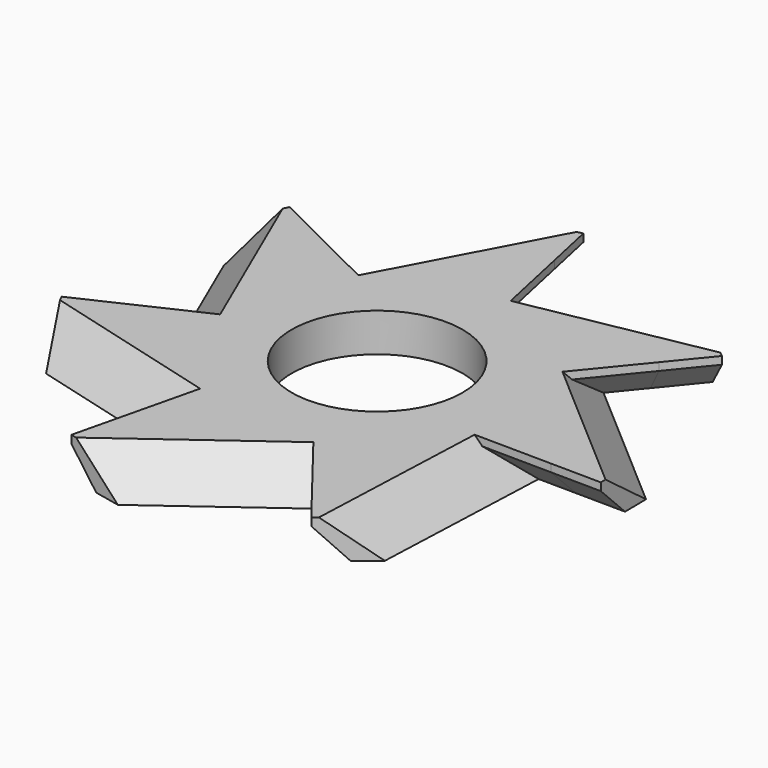
from build123d import *

# Parameters (mm, degrees)
F0_R         = 11.1
F1_DEPTH     = 5
F2_T4_DEPTH  = 66.9224244324
F2_T10_DEPTH = 66.9224244324
F2_T16_DEPTH = 66.9224244324
F2_T22_DEPTH = 66.9224244324
F2_T28_DEPTH = 66.9224244324
F2_T34_DEPTH = 66.9224244324
F2_T40_DEPTH = 66.9224244324
F3_SIZE      = 4


# Not quite as in the source:
# - a fillet or chamfer that OpenCascade refuses, or shapes differently, is made with other operations: its cross-section is extruded or revolved along the edge and cut away or added


with BuildPart() as f1:
    # F0 (on Top) → F1 (new body)
    with BuildSketch(Plane.XY):
        with BuildLine():
            ThreePointArc((13.9102940248, -6.3947663514), (14.9558155311, -3.2730564225), (15.3097784616, 0))
            ThreePointArc((15.3097784616, 0), (14.9174264356, 3.4437922532), (13.7604803953, 6.7110726292))
            ThreePointArc((13.7604803953, 6.7110726292), (13.7168049275, 6.7998955231), (13.6725561219, 6.8884341936))
            ThreePointArc((13.6725561219, 6.8884341936), (9.4080501116, 12.077992782), (3.3325913325, 14.9426621308))
            ThreePointArc((3.3325913325, 14.9426621308), (3.2359155889, 14.9638954436), (3.1391045899, 14.9845032923))
            ThreePointArc((3.1391045899, 14.9845032923), (-3.577131702, 14.8860150924), (-9.6048069761, 11.9221222731))
            ThreePointArc((-9.6048069761, 11.9221222731), (-9.6816841888, 11.8597768872), (-9.7581567243, 11.7969357838))
            ThreePointArc((-9.7581567243, 11.7969357838), (-13.8686603838, 6.4845644188), (-15.3095897294, -0.0760188232))
            ThreePointArc((-15.3095897294, -0.0760188232), (-15.308778302, -0.1749955606), (-15.307326995, -0.2739649836))
            ThreePointArc((-15.307326995, -0.2739649836), (-13.7168049275, -6.7998955231), (-9.4859391577, -12.0169161951))
            ThreePointArc((-9.4859391577, -12.0169161951), (-9.4080501116, -12.077992782), (-9.3297678259, -12.1385645305))
            ThreePointArc((-9.3297678259, -12.1385645305), (-3.2359155889, -14.9638954436), (3.4808170776, -14.9088305717))
            ThreePointArc((3.4808170776, -14.9088305717), (3.577131702, -14.8860150924), (3.6732968087, -14.8625774043))
            ThreePointArc((3.6732968087, -14.8625774043), (9.6816841888, -11.8597768872), (13.8264470578, -6.5740914431))
            ThreePointArc((13.8264470578, -6.5740914431), (13.8686603838, -6.4845644188), (13.9102940248, -6.3947663514))
        make_face()
        Circle(F0_R, mode=Mode.SUBTRACT)
        with BuildLine():
            ThreePointArc((13.6725561219, 6.8884341936), (13.7168049275, 6.7998955231), (13.7604803953, 6.7110726292))
            Line((13.7604803953, 6.7110726292), (28.1393743339, 1.1806929027))
            Line((28.1393743339, 1.1806929027), (27.8254993307, -6.5534854768))
            Line((27.8254993307, -6.5534854768), (34.3666750494, -6.6280952053))
            Line((34.3666750494, -6.6280952053), (34.1806906403, 7.5286378152))
            Line((34.1806906403, 7.5286378152), (22.47263633, 17.6688200307))
            Line((22.47263633, 17.6688200307), (13.6725561219, 6.8884341936))
        make_face()
        with BuildLine():
            ThreePointArc((13.7604803953, 6.7110726292), (14.9174264356, 3.4437922532), (15.3097784616, 0))
            ThreePointArc((15.3097784616, 0), (14.9558155311, -3.2730564225), (13.9102940248, -6.3947663514))
            Line((13.9102940248, -6.3947663514), (27.8254993307, -6.5534854768))
            Line((27.8254993307, -6.5534854768), (28.1393743339, 1.1806929027))
            Line((28.1393743339, 1.1806929027), (13.7604803953, 6.7110726292))
        make_face()
        with BuildLine():
            Line((27.8254993307, -6.5534854768), (13.9102940248, -6.3947663514))
            ThreePointArc((13.9102940248, -6.3947663514), (13.8686603838, -6.4845644188), (13.8264470578, -6.5740914431))
            Line((13.8264470578, -6.5740914431), (18.4677158103, -21.2640987672))
            Line((18.4677158103, -21.2640987672), (12.2251937987, -25.8408827536))
            Line((12.2251937987, -25.8408827536), (16.2452179168, -31.0014982676))
            Line((16.2452179168, -31.0014982676), (27.1974380987, -22.0295111355))
            Line((27.1974380987, -22.0295111355), (27.8254993307, -6.5534854768))
        make_face()
        with BuildLine():
            Line((18.4677158103, -21.2640987672), (13.8264470578, -6.5740914431))
            ThreePointArc((13.8264470578, -6.5740914431), (9.6816841888, -11.8597768872), (3.6732968087, -14.8625774043))
            Line((3.6732968087, -14.8625774043), (12.2251937987, -25.8408827536))
            Line((12.2251937987, -25.8408827536), (18.4677158103, -21.2640987672))
        make_face()
        with BuildLine():
            Line((12.2251937987, -25.8408827536), (3.6732968087, -14.8625774043))
            ThreePointArc((3.6732968087, -14.8625774043), (3.577131702, -14.8860150924), (3.4808170776, -14.9088305717))
            Line((3.4808170776, -14.9088305717), (-5.1105093912, -27.6965903568))
            Line((-5.1105093912, -27.6965903568), (-12.5809320123, -25.669568259))
            Line((-12.5809320123, -25.669568259), (-14.1092196492, -32.0301408191))
            Line((-14.1092196492, -32.0301408191), (-0.2660400579, -34.9989888809))
            Line((-0.2660400579, -34.9989888809), (12.2251937987, -25.8408827536))
        make_face()
        with BuildLine():
            Line((-5.1105093912, -27.6965903568), (3.4808170776, -14.9088305717))
            ThreePointArc((3.4808170776, -14.9088305717), (-3.2359155889, -14.9638954436), (-9.3297678259, -12.1385645305))
            Line((-9.3297678259, -12.1385645305), (-12.5809320123, -25.669568259))
            Line((-12.5809320123, -25.669568259), (-5.1105093912, -27.6965903568))
        make_face()
        with BuildLine():
            Line((-12.5809320123, -25.669568259), (-9.3297678259, -12.1385645305))
            ThreePointArc((-9.3297678259, -12.1385645305), (-9.4080501116, -12.077992782), (-9.4859391577, -12.0169161951))
            Line((-9.4859391577, -12.0169161951), (-24.8404167857, -13.2729845003))
            Line((-24.8404167857, -13.2729845003), (-27.9133594138, -6.1685453016))
            Line((-27.9133594138, -6.1685453016), (-33.8391270437, -8.939434038))
            Line((-33.8391270437, -8.939434038), (-27.5291846246, -21.6135141498))
            Line((-27.5291846246, -21.6135141498), (-12.5809320123, -25.669568259))
        make_face()
        with BuildLine():
            ThreePointArc((-15.307326995, -0.2739649836), (-15.308778302, -0.1749955606), (-15.3095897294, -0.0760188232))
            Line((-15.3095897294, -0.0760188232), (-25.8649836884, 11.1454494045))
            Line((-25.8649836884, 11.1454494045), (-22.2264578479, 17.9775180833))
            Line((-22.2264578479, 17.9775180833), (-28.0874815819, 20.8828489049))
            Line((-28.0874815819, 20.8828489049), (-34.062291676, 8.0473775715))
            Line((-34.062291676, 8.0473775715), (-27.9133594138, -6.1685453016))
            Line((-27.9133594138, -6.1685453016), (-15.307326995, -0.2739649836))
        make_face()
        with BuildLine():
            ThreePointArc((-15.3095897294, -0.0760188232), (-13.8686603838, 6.4845644188), (-9.7581567243, 11.7969357838))
            Line((-9.7581567243, 11.7969357838), (-22.2264578479, 17.9775180833))
            Line((-22.2264578479, 17.9775180833), (-25.8649836884, 11.1454494045))
            Line((-25.8649836884, 11.1454494045), (-15.3095897294, -0.0760188232))
        make_face()
        with BuildLine():
            ThreePointArc((-9.7581567243, 11.7969357838), (-9.6816841888, 11.8597768872), (-9.6048069761, 11.9221222731))
            Line((-9.6048069761, 11.9221222731), (-7.4126903243, 27.171132582))
            Line((-7.4126903243, 27.171132582), (0.1974198146, 28.5861436769))
            Line((0.1974198146, 28.5861436769), (-1.1853896087, 34.97992069))
            Line((-1.1853896087, 34.97992069), (-14.9457983513, 31.6484298448))
            Line((-14.9457983513, 31.6484298448), (-22.2264578479, 17.9775180833))
            Line((-22.2264578479, 17.9775180833), (-9.7581567243, 11.7969357838))
        make_face()
        with BuildLine():
            ThreePointArc((-9.6048069761, 11.9221222731), (-3.577131702, 14.8860150924), (3.1391045899, 14.9845032923))
            Line((3.1391045899, 14.9845032923), (0.1974198146, 28.5861436769))
            Line((0.1974198146, 28.5861436769), (-7.4126903243, 27.171132582))
            Line((-7.4126903243, 27.171132582), (-9.6048069761, 11.9221222731))
        make_face()
        with BuildLine():
            ThreePointArc((3.1391045899, 14.9845032923), (3.2359155889, 14.9638954436), (3.3325913325, 14.9426621308))
            Line((3.3325913325, 14.9426621308), (16.6215100454, 22.7363987351))
            Line((16.6215100454, 22.7363987351), (22.47263633, 17.6688200307))
            Line((22.47263633, 17.6688200307), (26.6093249174, 22.7363987351))
            Line((26.6093249174, 22.7363987351), (15.4251859707, 31.4175689347))
            Line((15.4251859707, 31.4175689347), (0.1974198146, 28.5861436769))
            Line((0.1974198146, 28.5861436769), (3.1391045899, 14.9845032923))
        make_face()
        with BuildLine():
            ThreePointArc((3.3325913325, 14.9426621308), (9.4080501116, 12.077992782), (13.6725561219, 6.8884341936))
            Line((13.6725561219, 6.8884341936), (22.47263633, 17.6688200307))
            Line((22.47263633, 17.6688200307), (16.6215100454, 22.7363987351))
            Line((16.6215100454, 22.7363987351), (3.3325913325, 14.9426621308))
        make_face()
        with BuildLine():
            Line((-24.8404167857, -13.2729845003), (-9.4859391577, -12.0169161951))
            ThreePointArc((-9.4859391577, -12.0169161951), (-13.7168049275, -6.7998955231), (-15.307326995, -0.2739649836))
            Line((-15.307326995, -0.2739649836), (-27.9133594138, -6.1685453016))
            Line((-27.9133594138, -6.1685453016), (-24.8404167857, -13.2729845003))
        make_face()
    extrude(amount=F1_DEPTH)

    # F2: chamfer of 10 on 7 edges, made by hand


with BuildPart() as f2_tool2:
    # F2_s3 → F2_t4 (new body)
    with BuildSketch(Plane(origin=(-1.8906345765, -46.5870327993, 0), x_dir=(0, 0, 1), z_dir=(0.0405494722, 0.9991775319, 0))):
        with BuildLine():
            Line((-5.2828427125, 28.3511968353), (5.2828427125, 17.7855114104))
            Line((5.2828427125, 17.7855114104), (5.4828427125, 17.7855114104))
            ThreePointArc((5.4828427125, 17.7855114104), (5.2, 22.9269327666), (5.2, 28.0683541229))
            Line((5.2, 28.0683541229), (5, 28.2683541229))
            ThreePointArc((5, 28.2683541229), (-0.1414213562, 28.2683541229), (-5.2828427125, 28.5511968353))
            Line((-5.2828427125, 28.5511968353), (-5.2828427125, 28.3511968353))
        make_face()
    extrude(amount=F2_T4_DEPTH)

    split(bisect_by=Plane(origin=(21.7213280078, -26.5155047015, 0), x_dir=(0, 0, 1), z_dir=(-0.6337064464, 0.7735736163, 0)), keep=Keep.TOP)

    split(bisect_by=Plane(origin=(-0.0711207687, -6.2352920297, 0), x_dir=(0, 0, 1), z_dir=(-0.0114054229, -0.999934956, 0)), keep=Keep.TOP)


with BuildPart() as f1_1:
    add(f1.part)

    # F2_t1: cut F2_tool2
    add(f2_tool2.part, mode=Mode.SUBTRACT)


with BuildPart() as f2_tool8:
    # F2_s9 → F2_t10 (new body)
    with BuildSketch(Plane(origin=(-37.6020002947, -27.5683822155, 0), x_dir=(0, 0, 1), z_dir=(0.8064706334, 0.5912741475, 0))):
        with BuildLine():
            Line((-5.2828427125, 28.3511968353), (5.2828427125, 17.7855114104))
            Line((5.2828427125, 17.7855114104), (5.4828427125, 17.7855114104))
            ThreePointArc((5.4828427125, 17.7855114104), (5.2, 22.9269327666), (5.2, 28.0683541229))
            Line((5.2, 28.0683541229), (5, 28.2683541229))
            ThreePointArc((5, 28.2683541229), (-0.1414213562, 28.2683541229), (-5.2828427125, 28.5511968353))
            Line((-5.2828427125, 28.5511968353), (-5.2828427125, 28.3511968353))
        make_face()
    extrude(amount=F2_T10_DEPTH)

    split(bisect_by=Plane(origin=(-7.1876298535, -33.51456485, 0), x_dir=(0, 0, 1), z_dir=(0.2096947006, 0.9777669112, 0)), keep=Keep.TOP)

    split(bisect_by=Plane(origin=(-4.9192906851, -3.8320365361, 0), x_dir=(0, 0, 1), z_dir=(-0.7888917939, -0.6145321289, 0)), keep=Keep.TOP)


with BuildPart() as f1_2:
    add(f1_1.part)

    # F2_t7: cut F2_tool8
    add(f2_tool8.part, mode=Mode.SUBTRACT)


with BuildPart() as f2_tool14:
    # F2_s15 → F2_t16 (new body)
    with BuildSketch(Plane(origin=(-44.99829285, 12.2098224691, 0), x_dir=(0, 0, 1), z_dir=(0.9651029587, -0.2618707298, 0))):
        with BuildLine():
            Line((-5.2828427125, 28.3511968353), (5.2828427125, 17.7855114104))
            Line((5.2828427125, 17.7855114104), (5.4828427125, 17.7855114104))
            ThreePointArc((5.4828427125, 17.7855114104), (5.2, 22.9269327666), (5.2, 28.0683541229))
            Line((5.2, 28.0683541229), (5, 28.2683541229))
            ThreePointArc((5, 28.2683541229), (-0.1414213562, 28.2683541229), (-5.2828427125, 28.5511968353))
            Line((-5.2828427125, 28.5511968353), (-5.2828427125, 28.3511968353))
        make_face()
    extrude(amount=F2_T16_DEPTH)

    split(bisect_by=Plane(origin=(-30.6841558342, -15.2764740939, 0), x_dir=(0, 0, 1), z_dir=(0.895191461, 0.4456817791, 0)), keep=Keep.TOP)

    split(bisect_by=Plane(origin=(-6.0631343805, 1.4568206285, 0), x_dir=(0, 0, 1), z_dir=(-0.9723265537, 0.2336259255, 0)), keep=Keep.TOP)


with BuildPart() as f1_3:
    add(f1_2.part)

    # F2_t13: cut F2_tool14
    add(f2_tool14.part, mode=Mode.SUBTRACT)


with BuildPart() as f2_tool20:
    # F2_s21 → F2_t22 (new body)
    with BuildSketch(Plane(origin=(-18.5099530914, 42.7937817994, 0), x_dir=(0, 0, 1), z_dir=(0.3969930716, -0.9178216064, 0))):
        with BuildLine():
            Line((-5.2828427125, 28.3511968353), (5.2828427125, 17.7855114104))
            Line((5.2828427125, 17.7855114104), (5.4828427125, 17.7855114104))
            ThreePointArc((5.4828427125, 17.7855114104), (5.2, 22.9269327666), (5.2, 28.0683541229))
            Line((5.2, 28.0683541229), (5, 28.2683541229))
            ThreePointArc((5, 28.2683541229), (-0.1414213562, 28.2683541229), (-5.2828427125, 28.5511968353))
            Line((-5.2828427125, 28.5511968353), (-5.2828427125, 28.3511968353))
        make_face()
    extrude(amount=F2_T22_DEPTH)

    split(bisect_by=Plane(origin=(-31.074886629, 14.4651132382, 0), x_dir=(0, 0, 1), z_dir=(0.9065907927, -0.4220108229, 0)), keep=Keep.TOP)

    split(bisect_by=Plane(origin=(-2.6413142219, 5.6486621461, 0), x_dir=(0, 0, 1), z_dir=(-0.4235795866, 0.9058588929, 0)), keep=Keep.TOP)


with BuildPart() as f1_4:
    add(f1_3.part)

    # F2_t19: cut F2_tool20
    add(f2_tool20.part, mode=Mode.SUBTRACT)


with BuildPart() as f2_tool26:
    # F2_s27 → F2_t28 (new body)
    with BuildSketch(Plane(origin=(21.9167588793, 41.1531506007, 0), x_dir=(0, 0, 1), z_dir=(-0.4700606956, -0.8826340932, 0))):
        with BuildLine():
            Line((-5.2828427125, 28.3511968353), (5.2828427125, 17.7855114104))
            Line((5.2828427125, 17.7855114104), (5.4828427125, 17.7855114104))
            ThreePointArc((5.4828427125, 17.7855114104), (5.2, 22.9269327666), (5.2, 28.0683541229))
            Line((5.2, 28.0683541229), (5, 28.2683541229))
            ThreePointArc((5, 28.2683541229), (-0.1414213562, 28.2683541229), (-5.2828427125, 28.5511968353))
            Line((-5.2828427125, 28.5511968353), (-5.2828427125, 28.3511968353))
        make_face()
    extrude(amount=F2_T28_DEPTH)

    split(bisect_by=Plane(origin=(-8.06559398, 33.3141752674, 0), x_dir=(0, 0, 1), z_dir=(0.2353087664, -0.9719206678, 0)), keep=Keep.TOP)

    split(bisect_by=Plane(origin=(2.7694694188, 5.586945856, 0), x_dir=(0, 0, 1), z_dir=(0.4441314486, 0.8959616378, 0)), keep=Keep.TOP)


with BuildPart() as f1_5:
    add(f1_4.part)

    # F2_t25: cut F2_tool26
    add(f2_tool26.part, mode=Mode.SUBTRACT)


with BuildPart() as f2_tool32:
    # F2_s33 → F2_t34 (new body)
    with BuildSketch(Plane(origin=(45.8397043935, 8.5233576284, 0), x_dir=(0, 0, 1), z_dir=(-0.9831491715, -0.1828051054, 0))):
        with BuildLine():
            Line((-5.2828427125, 28.3511968353), (5.2828427125, 17.7855114104))
            Line((5.2828427125, 17.7855114104), (5.4828427125, 17.7855114104))
            ThreePointArc((5.4828427125, 17.7855114104), (5.2, 22.9269327666), (5.2, 28.0683541229))
            Line((5.2, 28.0683541229), (5, 28.2683541229))
            ThreePointArc((5, 28.2683541229), (-0.1414213562, 28.2683541229), (-5.2828427125, 28.5511968353))
            Line((-5.2828427125, 28.5511968353), (-5.2828427125, 28.3511968353))
        make_face()
    extrude(amount=F2_T34_DEPTH)

    split(bisect_by=Plane(origin=(21.017255444, 27.0769838349, 0), x_dir=(0, 0, 1), z_dir=(-0.6131655604, -0.7899544263, 0)), keep=Keep.TOP)

    split(bisect_by=Plane(origin=(6.0947861002, 1.3181453834, 0), x_dir=(0, 0, 1), z_dir=(0.9774024444, 0.2113869951, 0)), keep=Keep.TOP)


with BuildPart() as f1_6:
    add(f1_5.part)

    # F2_t31: cut F2_tool32
    add(f2_tool32.part, mode=Mode.SUBTRACT)


with BuildPart() as f2_tool38:
    # F2_s39 → F2_t40 (new body)
    with BuildSketch(Plane(origin=(35.2444175398, -30.5246974829, 0), x_dir=(0, 0, 1), z_dir=(-0.7559062687, 0.6546798553, 0))):
        with BuildLine():
            Line((-5.2828427125, 28.3511968353), (5.2828427125, 17.7855114104))
            Line((5.2828427125, 17.7855114104), (5.4828427125, 17.7855114104))
            ThreePointArc((5.4828427125, 17.7855114104), (5.2, 22.9269327666), (5.2, 28.0683541229))
            Line((5.2, 28.0683541229), (5, 28.2683541229))
            ThreePointArc((5, 28.2683541229), (-0.1414213562, 28.2683541229), (-5.2828427125, 28.5511968353))
            Line((-5.2828427125, 28.5511968353), (-5.2828427125, 28.3511968353))
        make_face()
    extrude(amount=F2_T40_DEPTH)

    split(bisect_by=Plane(origin=(34.2736828448, 0.4502713049, 0), x_dir=(0, 0, 1), z_dir=(-0.9999137139, -0.0131363897, 0)), keep=Keep.TOP)

    split(bisect_by=Plane(origin=(4.8306045372, -3.9432454481, 0), x_dir=(0, 0, 1), z_dir=(0.7746694642, -0.6323663663, 0)), keep=Keep.TOP)


with BuildPart() as f1_7:
    add(f1_6.part)

    # F2_t37: cut F2_tool38
    add(f2_tool38.part, mode=Mode.SUBTRACT)

    # F3
    f3_edges = [f1_7.edges().sort_by_distance(p)[0] for p in [
        (22.959393, 18.265112, 0),
        (28.595187, -6.562265, 0),
        (12.698222, -26.448123, 0),
        (-12.760763, -26.418005, 0),
        (-28.610633, -6.49459, 0),
        (-22.916113, 18.319383, 0),
        (0.034707, 29.338487, 0),
    ]]
    chamfer(f3_edges, length=F3_SIZE)


solid = f1_7.part
